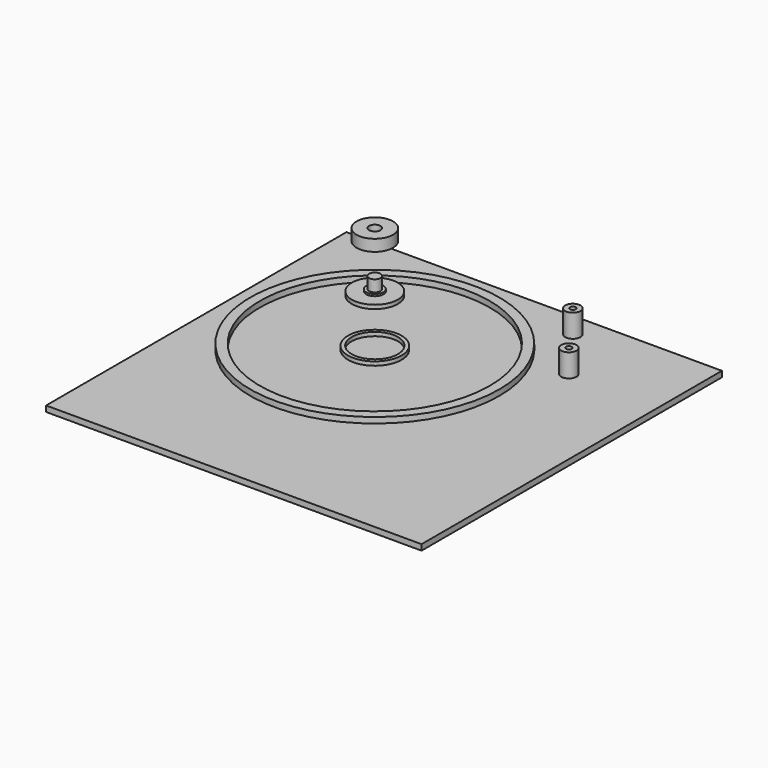
from build123d import *

# Parameters (mm, degrees)
F0_W      = 196
F0_H      = 196
F0_R      = 65
F0_R_2    = 4
F0_R_3    = 60
F0_R_4    = 14
F0_R_5    = 12.1
F1_DEPTH  = 3
F0_R_6    = 1.5
F2_DEPTH  = 15
F4_R      = 12
F4_R_2    = 4.5
F5_DEPTH  = 2
F4_R_3    = 3
F6_DEPTH  = 3
F7_DEPTH  = 9
F8_DEPTH  = 5
F10_R     = 9.5
F10_R_2   = 3
F11_DEPTH = 6
F12_DEPTH = 6


# Not quite as in the source:
# - a feature names something its author has since deleted; it is built from what else it names


with BuildPart() as f1:
    # F0 (on Top) → F1 (new body)
    with BuildSketch(Plane.XY):
        Rectangle(F0_W, F0_H)
        with Locations((-24, 24)):
            Circle(F0_R, mode=Mode.SUBTRACT)
        with Locations((30.4351176349, 85.180617585)):
            Circle(F0_R_2, mode=Mode.SUBTRACT)
        with Locations((51.0076014651, 56.8650227818)):
            Circle(F0_R_2, mode=Mode.SUBTRACT)
        with Locations((-24, 24)):
            Circle(F0_R)
        with Locations((-24, 24)):
            Circle(F0_R_3, mode=Mode.SUBTRACT)
        with Locations((-24, 24)):
            Circle(F0_R_3)
        with Locations((-24, 24)):
            Circle(F0_R_4, mode=Mode.SUBTRACT)
        with Locations((-24, 24)):
            Circle(F0_R_4)
        with Locations((-24, 24)):
            Circle(F0_R_5, mode=Mode.SUBTRACT)
        with Locations((-24, 24)):
            Circle(F0_R_5)
    extrude(amount=F1_DEPTH)

    # F0 (on Top) → F2 (join)
    with BuildSketch(Plane.XY):
        with Locations((30.4351176349, 85.180617585)):
            Circle(F0_R_2)
        with Locations((30.4351176349, 85.180617585)):
            Circle(F0_R_6, mode=Mode.SUBTRACT)
        with Locations((51.0076014651, 56.8650227818)):
            Circle(F0_R_2)
        with Locations((51.0076014651, 56.8650227818)):
            Circle(F0_R_6, mode=Mode.SUBTRACT)
    extrude(amount=F2_DEPTH)

    # F0 (on Top) → F8 (join)
    with BuildSketch(Plane.XY):
        with Locations((-24, 24)):
            Circle(F0_R_4)
        with Locations((-24, 24)):
            Circle(F0_R_5, mode=Mode.SUBTRACT)
    extrude(amount=F8_DEPTH)

    # F0 (on Top) → F12 (join)
    with BuildSketch(Plane.XY):
        with Locations((-24, 24)):
            Circle(F0_R)
        with Locations((-24, 24)):
            Circle(F0_R_3, mode=Mode.SUBTRACT)
    extrude(amount=F12_DEPTH)


with BuildPart() as f5:
    # F4 (on offset) → F5 (new body)
    with BuildSketch(Plane.XY.offset(28)):
        with Locations((-24, 24)):
            Circle(F4_R)
        with Locations((-24, 24)):
            Circle(F4_R_2, mode=Mode.SUBTRACT)
    extrude(amount=F5_DEPTH)

    # F4 (on offset) → F6 (join)
    with BuildSketch(Plane.XY.offset(28)):
        with Locations((-24, 24)):
            Circle(F4_R_2)
        with Locations((-24, 24)):
            Circle(F4_R_3, mode=Mode.SUBTRACT)
    extrude(amount=F6_DEPTH)

    # F4 (on offset) → F7 (join)
    with BuildSketch(Plane.XY.offset(28)):
        with Locations((-24, 24)):
            Circle(F4_R_3)
    extrude(amount=F7_DEPTH)


with BuildPart() as f11:
    # F10 (on offset) → F11 (new body)
    with BuildSketch(Plane.XY.offset(53)):
        with Locations((-24, 24)):
            Circle(F10_R)
        with Locations((-24, 24)):
            Circle(F10_R_2, mode=Mode.SUBTRACT)
    extrude(amount=F11_DEPTH)


solid = Compound([f1.part, f5.part, f11.part])
